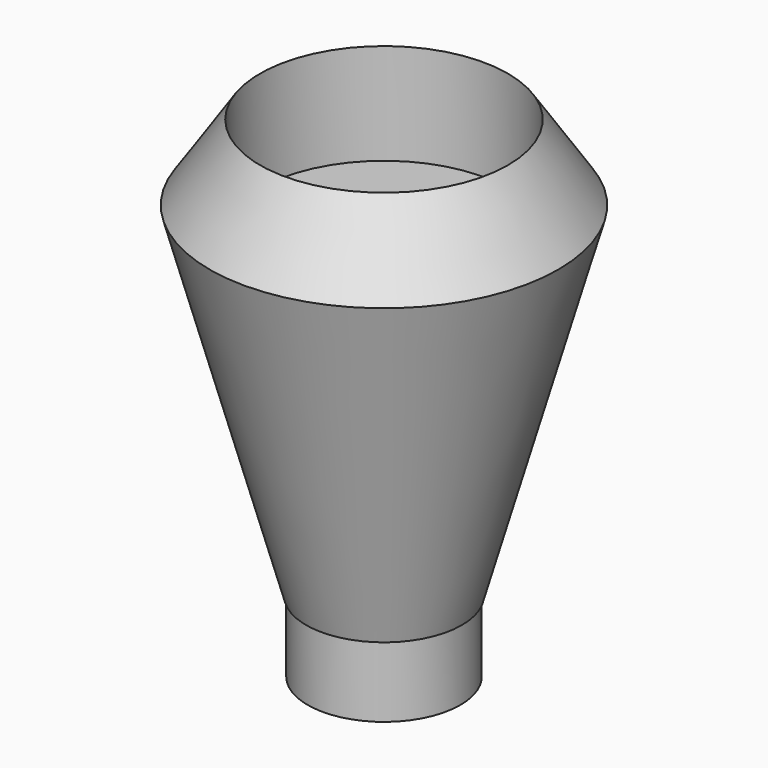
from build123d import *

# Parameters (mm, degrees)
F0_R     = 15.875
F1_DEPTH = 31.75
F2_R     = 6.8433299252
F3_DEPTH = 6.35
F4_DEPTH = 6.35
F5_R     = 11.1125
F6_DEPTH = 9.525
F7_R     = 4.7625
F8_DEPTH = 25.4
F9_SIZE2 = 8.89
F9_SIZE  = 31.75


# Not quite as in the source:
# - a fillet or chamfer that OpenCascade refuses, or shapes differently, is made with other operations: its cross-section is extruded or revolved along the edge and cut away or added


with BuildPart() as f1:
    # F0 (on Top) → F1 (new body)
    with BuildSketch(Plane.XY):
        Circle(F0_R)
    extrude(amount=F1_DEPTH)

    # F2 (on face) → F3 (join)
    with BuildSketch(Plane(origin=(0, 0, 0), x_dir=(1, 0, 0), z_dir=(0, 0, -1))):
        Circle(F2_R)
    extrude(amount=F3_DEPTH)

    # F4 (add): a face of the model
    f4_faces = [f1.faces().sort_by_distance(p)[0] for p in [
        (0, 0, 31.75),
    ]]
    extrude(f4_faces, amount=F4_DEPTH)

    # F5 (on face) → F6 (cut)
    with BuildSketch(Plane.XY.offset(38.1)):
        Circle(F5_R)
    extrude(amount=-F6_DEPTH, mode=Mode.SUBTRACT)

    # F7 (on face) → F8 (cut)
    with BuildSketch(Plane.XY.offset(28.575)):
        Circle(F7_R)
    extrude(amount=-F8_DEPTH, mode=Mode.SUBTRACT)

    # F9
    f9_edges = [f1.edges().sort_by_distance(p)[0] for p in [
        (-15.875, 0, 0),
    ]]
    f9_side = f1.faces().sort_by_distance((-15.875, 0, 19.05))[0]
    chamfer(f9_edges, length=F9_SIZE, length2=F9_SIZE2, reference=f9_side)

    # F10: chamfer of 5.08 x 7.62 on 1 edges, made by hand

    # F10_s1 → F10_t2 (revolve, cut)
    with BuildSketch(Plane.XZ):
        Polygon((15.875, 30.48), (10.795, 38.1), (15.875, 38.1), align=None)
    revolve(axis=Axis((0, 0, 38.1), (0, 0, 1)), mode=Mode.SUBTRACT)


solid = f1.part
